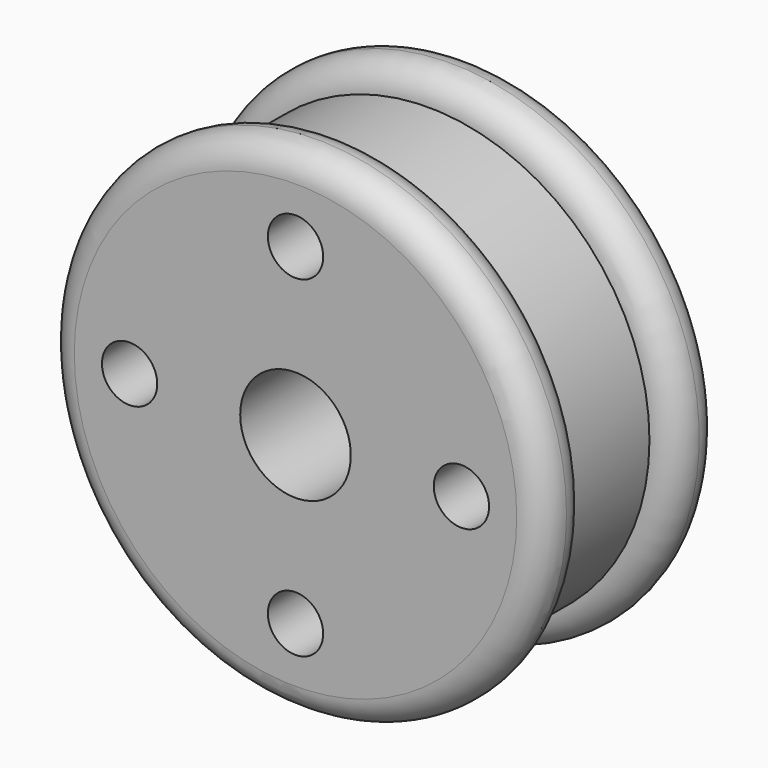
from build123d import *

# Parameters (mm, degrees)
F0_R     = 25.4
F1_DEPTH = 12.7
F2_R     = 28.575
F3_DEPTH = 6.35
F4_R     = 28.575
F5_DEPTH = 6.35
F6_R     = 6.35
F7_DEPTH = 25.401
F9_D     = 6.35
F10_R    = 3.17499


# Not quite as in the source:
# - a fillet or chamfer is up to 0.001 mm smaller than in the source, because OpenCascade refuses the exact size


with BuildPart() as f1:
    # F0 (on Front) → F1 (new body)
    with BuildSketch(Plane.XZ):
        Circle(F0_R)
    extrude(amount=F1_DEPTH)

    # F2 (on face) → F3 (join)
    with BuildSketch(Plane.XZ.offset(12.7)):
        Circle(F2_R)
    extrude(amount=F3_DEPTH)

    # F4 (on face) → F5 (join)
    with BuildSketch(Plane(origin=(0, 0, 0), x_dir=(-1, 0, 0), z_dir=(0, 1, 0))):
        Circle(F4_R)
    extrude(amount=F5_DEPTH)

    # F6 (on face) → F7 (cut, through all)
    with BuildSketch(Plane(origin=(0, 6.35, 0), x_dir=(-1, 0, 0), z_dir=(0, 1, 0))):
        Circle(F6_R)
    extrude(amount=-F7_DEPTH, mode=Mode.SUBTRACT)

    # F9 (through all)
    with Locations(Plane(origin=(0, 6.35, 0), x_dir=(-1, 0, 0), z_dir=(0, 1, 0))):
        with Locations((0, 19.05), (19.05, 0), (0, -19.05), (-19.05, 0)):
            Hole(F9_D / 2)

    # F10 (radius 3.175 in the source; OpenCascade refuses exactly that, so slightly less here)
    f10_edges = [f1.edges().sort_by_distance(p)[0] for p in [
        (28.575, 6.35, 0),
        (28.575, 0, 0),
        (-28.575, -12.7, 0),
        (-28.575, -19.05, 0),
    ]]
    fillet(f10_edges, radius=F10_R)


solid = f1.part
